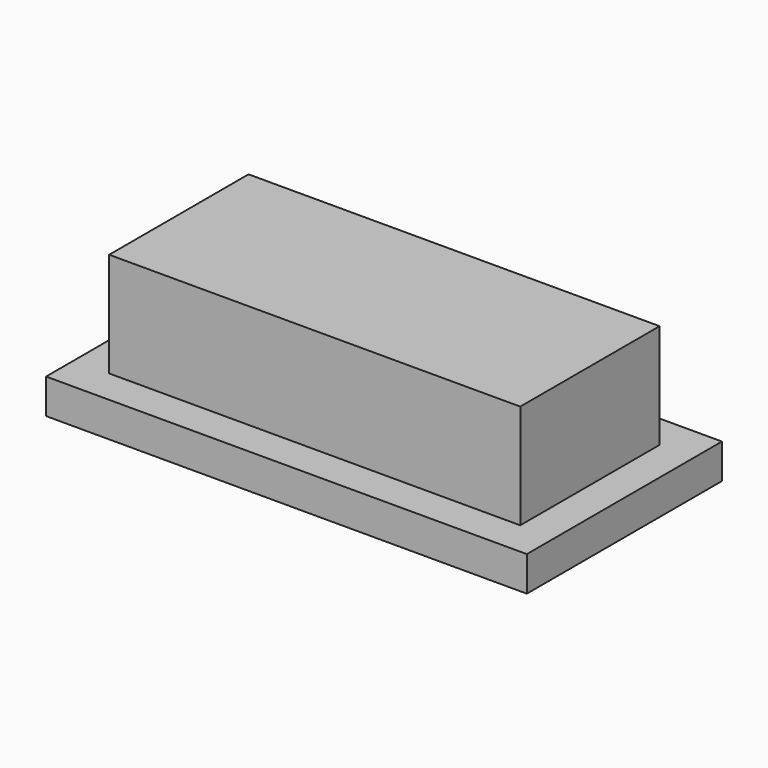
from build123d import *

# Parameters (mm, degrees)
F0_W     = 1380
F0_H     = 700
F0_W_2   = 1180
F0_H_2   = 500
F1_DEPTH = 100
F2_W     = 1180
F2_H     = 500
F3_DEPTH = 300
F4_R     = 55
F5_DEPTH = 1819
F6_DEPTH = 400.001
F8_DEPTH = 100


# Not quite as in the source:
# - an extrude ends at something that could not be found from the text; its depth is read off the source's solid
# - a feature of the source that left no trace in its solid (it failed there, or was rolled back) is left out


with BuildPart() as f1:
    # F0 (on Top) → F1 (new body)
    with BuildSketch(Plane.XY):
        Rectangle(F0_W, F0_H)
        Rectangle(F0_W_2, F0_H_2, mode=Mode.SUBTRACT)
        Rectangle(F0_W_2, F0_H_2)
    extrude(amount=F1_DEPTH)

    # F2 (on face) → F3 (join)
    with BuildSketch(Plane.XY.offset(100)):
        with Locations((1.1069327593, 0)):
            Rectangle(F2_W, F2_H)
    extrude(amount=F3_DEPTH)

    # F4 (on face) → F5 (cut, through all)
    with BuildSketch(Plane.XY.offset(400)):
        with BuildLine():
            ThreePointArc((-340, 150), (-490, 0), (-340, -150))
            Line((-340, -150), (340, -150))
            ThreePointArc((340, -150), (490, 0), (340, 150))
            Line((340, 150), (-340, 150))
        make_face()
        with Locations((-340, 0)):
            Circle(F4_R, mode=Mode.SUBTRACT)
        with Locations((340, 0)):
            Circle(F4_R, mode=Mode.SUBTRACT)
    extrude(amount=F5_DEPTH, mode=Mode.SUBTRACT)

    # F4 (on face) → F6 (cut, through all)
    with BuildSketch(Plane.XY.offset(400)):
        with BuildLine():
            ThreePointArc((-340, 150), (-490, 0), (-340, -150))
            Line((-340, -150), (340, -150))
            ThreePointArc((340, -150), (490, 0), (340, 150))
            Line((340, 150), (-340, 150))
        make_face()
        with Locations((-340, 0)):
            Circle(F4_R, mode=Mode.SUBTRACT)
        with Locations((340, 0)):
            Circle(F4_R, mode=Mode.SUBTRACT)
    extrude(amount=-F6_DEPTH, mode=Mode.SUBTRACT)

    # F4 (on face) → F8 (join)
    with BuildSketch(Plane.XY.offset(400)):
        with BuildLine():
            ThreePointArc((-340, 150), (-490, 0), (-340, -150))
            Line((-340, -150), (340, -150))
            ThreePointArc((340, -150), (490, 0), (340, 150))
            Line((340, 150), (-340, 150))
        make_face()
        with Locations((-340, 0)):
            Circle(F4_R, mode=Mode.SUBTRACT)
        with Locations((340, 0)):
            Circle(F4_R, mode=Mode.SUBTRACT)
        with Locations((-340, 0)):
            Circle(F4_R)
        with Locations((340, 0)):
            Circle(F4_R)
    extrude(amount=-F8_DEPTH)


solid = f1.part
